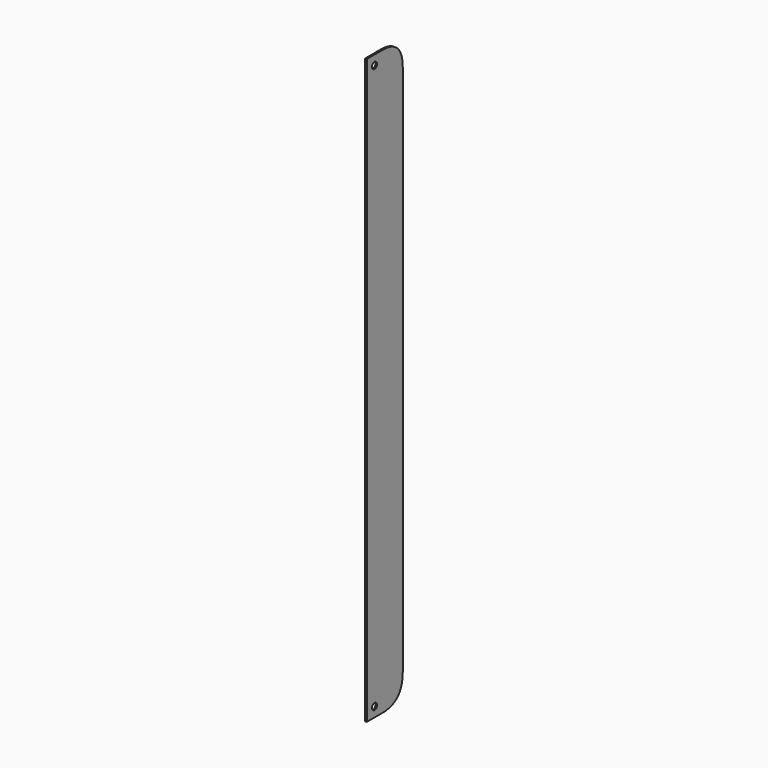
from build123d import *

# Parameters (mm, degrees)
F0_W        = 1.5875
F0_H        = 44.45
F1_DEPTH    = 577.85
F2_R        = 3.175
F3_DEPTH    = 1.5875
F4_T1_DEPTH = 128.5875


# Not quite as in the source:
# - a fillet or chamfer that OpenCascade refuses, or shapes differently, is made with other operations: its cross-section is extruded or revolved along the edge and cut away or added


with BuildPart() as f1:
    # F0 (on Top) → F1 (new body)
    with BuildSketch(Plane.XY):
        with Locations((-53.6594138073, 18.865058393)):
            Rectangle(F0_W, F0_H)
    extrude(amount=F1_DEPTH)

    # F2 (on face) → F3 (cut)
    with BuildSketch(Plane(origin=(-54.4531638073, 0, 0), x_dir=(0, -1, 0), z_dir=(-1, 0, 0))):
        with Locations((-6.165058393, 9.525)):
            Circle(F2_R)
        with Locations((-6.165058393, 568.325)):
            Circle(F2_R)
    extrude(amount=-F3_DEPTH, mode=Mode.SUBTRACT)

    # F4: fillet of radius 25.4 on 2 edges, made by hand

    # F4_s2 → F4_t1 (cut)
    with BuildSketch(Plane.YZ.offset(-117.9531638073)):
        with BuildLine():
            add(Edge.make_bspline(
                [(15.690058393, 577.85), (41.090058393, 577.85), (41.090058393, 552.45)],
                knots=[0, 0, 0, 1, 1, 1], degree=2, weights=[1, 1, 1]))
            Line((41.090058393, 552.45), (41.090058393, 577.85))
            Line((41.090058393, 577.85), (15.690058393, 577.85))
        make_face()
        with BuildLine():
            add(Edge.make_bspline(
                [(15.690058393, 0), (41.090058393, 0), (41.090058393, 25.4)],
                knots=[0, 0, 0, 1, 1, 1], degree=2, weights=[1, 1, 1]))
            Line((41.090058393, 25.4), (41.090058393, 0))
            Line((41.090058393, 0), (15.690058393, 0))
        make_face()
    extrude(amount=F4_T1_DEPTH, mode=Mode.SUBTRACT)


solid = f1.part
